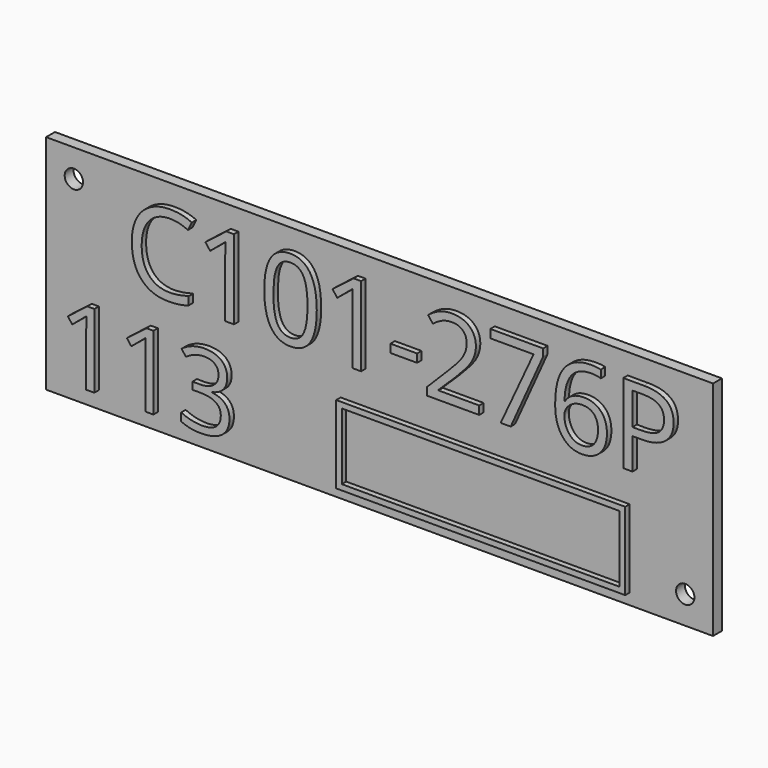
from build123d import *

# Parameters (mm, degrees)
F0_W         = 120
F0_H         = 40
F1_DEPTH     = 2
F3_D         = 3.3
F4_TEXT_SIZE = 20.0056265825
F5_DEPTH     = 1
F6_TEXT_SIZE = 18.5894526641
F7_DEPTH     = 1
F8_W         = 52
F8_H         = 14
F8_W_2       = 49.99999962
F8_H_2       = 11.99999962
F9_DEPTH     = 1


# Not quite as in the source:
# - Text() gives the source's letters only with a copy of the font that has no kerning and outlines rounded to 1/6400 em; it was checked with that copy


with BuildPart() as f1:
    # F0 (on Front) → F1 (new body)
    with BuildSketch(Plane.XZ):
        Rectangle(F0_W, F0_H)
    extrude(amount=F1_DEPTH)

    # F3 (through all)
    with Locations(Plane.XZ.offset(2)):
        with Locations((-55, 15), (55, -15)):
            Hole(F3_D / 2)

    # F4 (on face) → F5 (join)
    with BuildSketch(Plane.XZ.offset(2)):
        with Locations((-45, 2)):
            Text('C101-276P', F4_TEXT_SIZE, font='Open Sans', text_align=(TextAlign.LEFT, TextAlign.BOTTOM))
    extrude(amount=F5_DEPTH)

    # F6 (on face) → F7 (join)
    with BuildSketch(Plane.XZ.offset(2)):
        with Locations((-57, -17)):
            Text('113', F6_TEXT_SIZE, font='Open Sans', text_align=(TextAlign.LEFT, TextAlign.BOTTOM))
    extrude(amount=F7_DEPTH)

    # F8 (on face) → F9 (join)
    with BuildSketch(Plane.XZ.offset(2)):
        with Locations((19, -11)):
            Rectangle(F8_W, F8_H)
        with Locations((19, -11)):
            Rectangle(F8_W_2, F8_H_2, mode=Mode.SUBTRACT)
    extrude(amount=F9_DEPTH)


solid = f1.part
